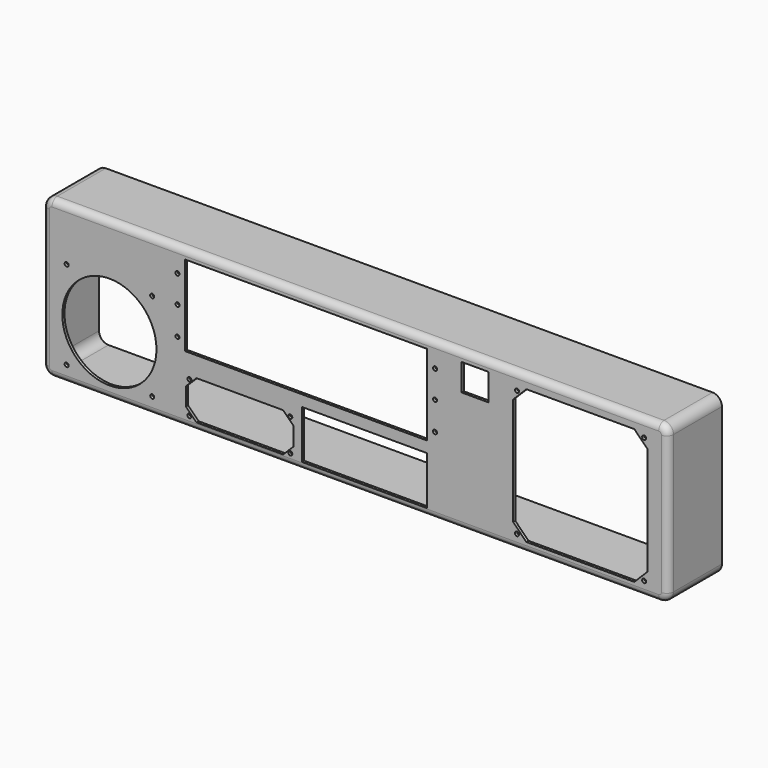
from build123d import *

# Parameters (mm, degrees)
F0_W     = 465
F0_H     = 117
F1_DEPTH = 50
F2_T     = -2
F4_R     = 7
F3_W     = 180
F3_H     = 60
F3_W_2   = 20
F3_H_2   = 20
F3_W_3   = 93
F3_H_3   = 36
F3_R     = 1.5
F3_W_4   = 77
F3_H_4   = 77
F3_R_2   = 9.5
F3_R_3   = 35
F5_DEPTH = 25
F6_R     = 5


with BuildPart() as f1:
    # F0 (on Front) → F1 (new body)
    with BuildSketch(Plane.XZ):
        with Locations((-12.6529467106, 27.1878533959)):
            Rectangle(F0_W, F0_H)
    extrude(amount=F1_DEPTH)

    # F2
    f2_openings = [f1.faces().sort_by_distance(p)[0] for p in [
        (-12.652947, 0, 27.187853),
    ]]
    offset(amount=F2_T, openings=f2_openings)

    # F4
    f4_edges = [f1.edges().sort_by_distance(p)[0] for p in [
        (-245.152947, -25, 85.687853),
        (219.847053, -25, 85.687853),
        (219.847053, -25, -31.312147),
        (-245.152947, -25, -31.312147),
        (-243.152947, -24, 83.687853),
        (-243.152947, -24, -29.312147),
        (217.847053, -24, -29.312147),
        (217.847053, -24, 83.687853),
    ]]
    fillet(f4_edges, radius=F4_R)

    # F3 (on face) → F5 (cut)
    with BuildSketch(Plane.XZ.offset(50)):
        with Locations((-49.312419115, 48.5197262004)):
            Rectangle(F3_W, F3_H)
        with Locations((76.3836680665, 68.3190373614)):
            Rectangle(F3_W_2, F3_H_2)
        Polygon((194.7213235501, 76.111191912), (114.5203134233, 76.111191912), (104.6208184867, 66.2116969754), (104.6208184867, -13.9893131514), (114.5203134233, -23.888808088), (194.7213235501, -23.888808088), (204.6208184867, -13.9893131514), (204.6208184867, 66.2116969754), align=None)
        with Locations((-81.5471372292, -73.4631650165)):
            Rectangle(F3_W_3, F3_H_3)
        with Locations((46.5855184052, 67.5480939005)):
            Circle(F3_R)
        with Locations((46.5855184052, 47.158148972)):
            Circle(F3_R)
        with Locations((46.5855184052, 26.052269754)):
            Circle(F3_R)
        with Locations((-195.3124095783, -98.1716645822)):
            Rectangle(F3_W_4, F3_H_4)
        with Locations((107.5167332374, 72.8625404379)):
            Circle(F3_R)
        with Locations((80.878779198, -82.3583360478)):
            Rectangle(F3_W_3, F3_H_3)
        with Locations((51.3206828289, -84.0745766136)):
            Circle(F3_R_2, mode=Mode.SUBTRACT)
        with Locations((81.3476530956, -84.0745766136)):
            Circle(F3_R_2, mode=Mode.SUBTRACT)
        with Locations((123.378779198, -96.3583360478)):
            Circle(F3_R, mode=Mode.SUBTRACT)
        with Locations((110.7360261029, -84.0745766136)):
            Circle(F3_R_2, mode=Mode.SUBTRACT)
        with Locations((38.378779198, -68.3583360478)):
            Circle(F3_R, mode=Mode.SUBTRACT)
        Polygon((-66.2842570873, 3.6055132091), (-130.7279079012, 3.6055132091), (-138.5060824942, -4.172661384), (-138.5060824942, -17.6163121979), (-130.7279079012, -25.3944867909), (-66.2842570873, -25.3944867909), (-58.5060824942, -17.6163121979), (-58.5060824942, -4.172661384), align=None)
        with Locations((-136.0060824942, 1.1055132091)):
            Circle(F3_R)
        with Locations((-136.0060824942, -22.8944867909)):
            Circle(F3_R)
        with Locations((-61.0060824942, 1.1055132091)):
            Circle(F3_R)
        with Locations((-61.0060824942, -22.8944867909)):
            Circle(F3_R)
        with Locations((107.5167332374, -20.8455865502)):
            Circle(F3_R)
        with Locations((202.0370356229, -20.8455660029)):
            Circle(F3_R)
        with Locations((202.0370356229, 72.8625404379)):
            Circle(F3_R)
        with Locations((-195.4793932134, 12.7347313118)):
            Circle(F3_R_3)
        with Locations((-144.8539147958, 67.5480939005)):
            Circle(F3_R)
        with Locations((-144.8539147958, 47.158148972)):
            Circle(F3_R)
        with Locations((-144.8539147958, 26.052269754)):
            Circle(F3_R)
        with Locations((-227.2830040105, 46.6578847659)):
            Circle(F3_R)
        with Locations((-227.2830040105, -19.1012599602)):
            Circle(F3_R)
        with Locations((-163.6415483004, -19.1012599602)):
            Circle(F3_R)
        with Locations((-5.8271809206, -7.7349814937)):
            Rectangle(F3_W_3, F3_H_3)
        with Locations((-163.6757824164, 46.6578847659)):
            Circle(F3_R)
    extrude(amount=-F5_DEPTH, mode=Mode.SUBTRACT)

    # F6
    f6_edges = [f1.edges().sort_by_distance(p)[0] for p in [
        (217.796801, -50, 83.637601),
    ]]
    fillet(f6_edges, radius=F6_R)


solid = f1.part
